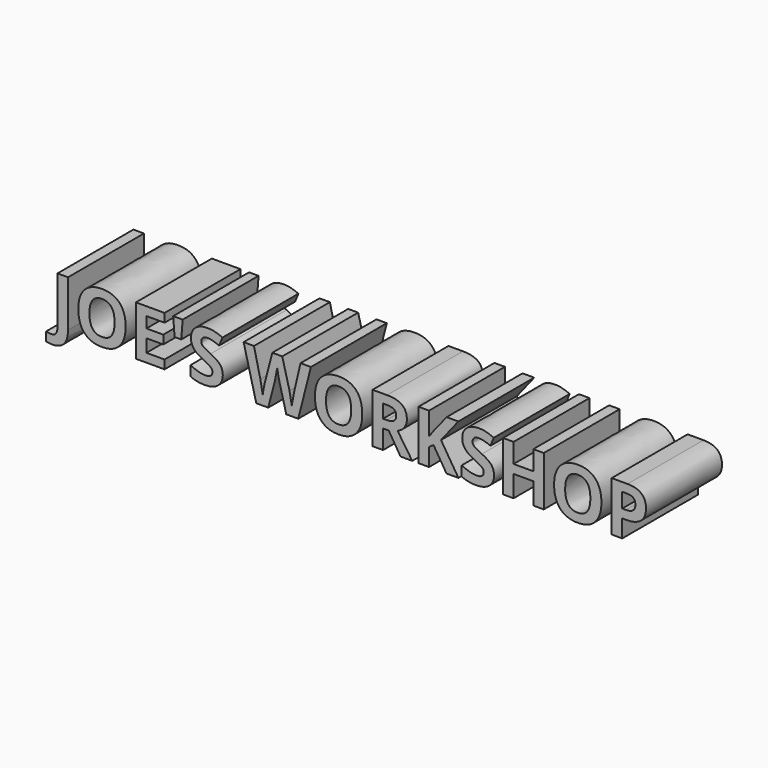
from build123d import *

# Parameters (mm, degrees)
F0_TEXT_SIZE = 18.6317341609
F1_DEPTH     = 25.4


# Not quite as in the source:
# - Text() gives the source's letters only with a copy of the font that has no kerning and outlines rounded to 1/6400 em; it was checked with that copy


with BuildPart() as f1:
    # F0 (on Front) → F1 (new body)
    with BuildSketch(Plane.XZ):
        with Locations((-98.159134388, 42.2440581024)):
            Text("JOE'S WORKSHOP", F0_TEXT_SIZE, font='Open Sans', font_style=FontStyle.BOLD, text_align=(TextAlign.LEFT, TextAlign.BOTTOM))
    extrude(amount=F1_DEPTH)


solid = f1.part
